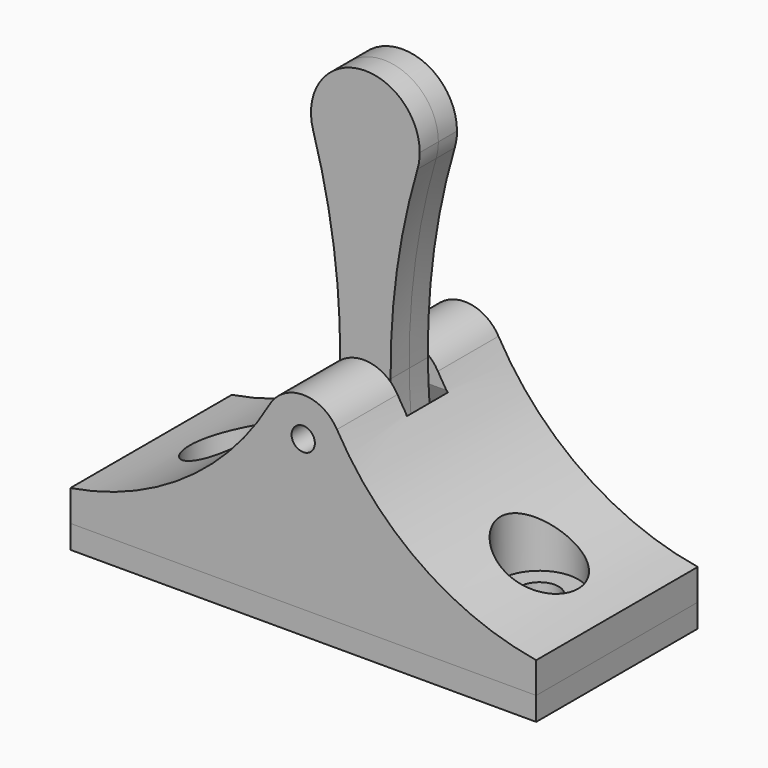
from build123d import *

# Parameters (mm, degrees)
F0_R          = 1.5
F1_DEPTH      = 3
F1_DEPTH_BACK = 3
F2_DEPTH      = 13
F2_DEPTH_BACK = 13
F3_W          = 11
F3_H          = 6.5
F4_DEPTH      = 25
F4_TAPER      = -22
F4_DEPTH_BACK = 25
F5_START      = -20
F3_W_2        = 60
F3_H_2        = 26
F3_R          = 5
F3_W_3        = 19
F3_H_3        = 13.5
F3_R_2        = 2.5
F5_DEPTH      = 3
F6_DEPTH      = 25
F7_DEPTH      = 17


# Not quite as in the source:
# - a feature names something its author has since deleted; it is built from what else it names


with BuildPart() as f1:
    # F0 (on Front) → F1 (new body, two sides)
    with BuildSketch(Plane.XZ) as f1_sk:
        with BuildLine():
            ThreePointArc((3.0397368307, -16), (4.3012352845, -14.3654093944), (4.75, -12.35))
            ThreePointArc((4.75, -12.35), (4.7300948444, -11.9156006874), (4.6705462051, -11.4848421267))
            ThreePointArc((4.6705462051, -11.4848421267), (0, -7.6), (-4.6705462051, -11.4848421267))
            ThreePointArc((-4.6705462051, -11.4848421267), (-4.4675249052, -13.9636050389), (-3.0397368307, -16))
            Line((-3.0397368307, -16), (3.0397368307, -16))
        make_face()
        with BuildLine():
            ThreePointArc((-4.6705462051, -11.4848421267), (0, -7.6), (4.6705462051, -11.4848421267))
            ThreePointArc((4.6705462051, -11.4848421267), (4.0724799807, -7.8080264222), (3.6360864347, -4.1085375916))
            ThreePointArc((3.6360864347, -4.1085375916), (0, -5.6765009603), (-3.6360864347, -4.1085375916))
            ThreePointArc((-3.6360864347, -4.1085375916), (-4.0724799807, -7.8080264222), (-4.6705462051, -11.4848421267))
        make_face()
        with BuildLine():
            ThreePointArc((-3.0397368307, -16), (0, -17.1), (3.0397368307, -16))
            Line((3.0397368307, -16), (-3.0397368307, -16))
        make_face()
        with BuildLine():
            ThreePointArc((-3.6360864347, -4.1085375916), (0, -5.6765009603), (3.6360864347, -4.1085375916))
            ThreePointArc((3.6360864347, -4.1085375916), (3.3676823781, -0.498156975), (3.2532612438, 3.1203781897))
            ThreePointArc((3.2532612438, 3.1203781897), (0, 4.3234990397), (-3.2532612438, 3.1203781897))
            ThreePointArc((-3.2532612438, 3.1203781897), (-3.3676823781, -0.498156975), (-3.6360864347, -4.1085375916))
        make_face()
        with Locations((0, -0.6765009603)):
            Circle(F0_R, mode=Mode.SUBTRACT)
        with BuildLine():
            ThreePointArc((-3.2532612438, 3.1203781897), (0, 4.3234990397), (3.2532612438, 3.1203781897))
            ThreePointArc((3.2532612438, 3.1203781897), (4.0582011416, 15.6996189973), (6.7145781542, 28.0215055695))
            ThreePointArc((6.7145781542, 28.0215055695), (0, 23), (-6.7145781542, 28.0215055695))
            ThreePointArc((-6.7145781542, 28.0215055695), (-4.0582011416, 15.6996189973), (-3.2532612438, 3.1203781897))
        make_face()
        with BuildLine():
            ThreePointArc((-6.7145781542, 28.0215055695), (0, 23), (6.7145781542, 28.0215055695))
            ThreePointArc((6.7145781542, 28.0215055695), (6.9282770975, 29.0005119008), (7, 30))
            ThreePointArc((7, 30), (-0.9994880992, 36.9282770975), (-6.7145781542, 28.0215055695))
        make_face()
    extrude(amount=F1_DEPTH)
    extrude(f1_sk.sketch, amount=-F1_DEPTH_BACK)


with BuildPart() as f2:
    # F0 (on Front) → F2 (new body, two sides)
    with BuildSketch(Plane.XZ) as f2_sk:
        with BuildLine():
            ThreePointArc((3.0397368307, -16), (4.3012352845, -14.3654093944), (4.75, -12.35))
            ThreePointArc((4.75, -12.35), (4.7300948444, -11.9156006874), (4.6705462051, -11.4848421267))
            ThreePointArc((4.6705462051, -11.4848421267), (0, -7.6), (-4.6705462051, -11.4848421267))
            ThreePointArc((-4.6705462051, -11.4848421267), (-4.4675249052, -13.9636050389), (-3.0397368307, -16))
            Line((-3.0397368307, -16), (3.0397368307, -16))
        make_face()
        with BuildLine():
            ThreePointArc((4.6705462051, -11.4848421267), (4.7300948444, -11.9156006874), (4.75, -12.35))
            ThreePointArc((4.75, -12.35), (4.3012352845, -14.3654093944), (3.0397368307, -16))
            Line((3.0397368307, -16), (30, -16))
            ThreePointArc((30, -16), (15.1577815574, -9.9967996829), (4.3401298873, 1.8060929577))
            ThreePointArc((4.3401298873, 1.8060929577), (4.8322173708, 0.607895895), (5, -0.6765009603))
            ThreePointArc((5, -0.6765009603), (4.6465273148, -2.5230609818), (3.6360864347, -4.1085375916))
            ThreePointArc((3.6360864347, -4.1085375916), (4.0724799807, -7.8080264222), (4.6705462051, -11.4848421267))
        make_face()
        with BuildLine():
            ThreePointArc((-4.6705462051, -11.4848421267), (0, -7.6), (4.6705462051, -11.4848421267))
            ThreePointArc((4.6705462051, -11.4848421267), (4.0724799807, -7.8080264222), (3.6360864347, -4.1085375916))
            ThreePointArc((3.6360864347, -4.1085375916), (0, -5.6765009603), (-3.6360864347, -4.1085375916))
            ThreePointArc((-3.6360864347, -4.1085375916), (-4.0724799807, -7.8080264222), (-4.6705462051, -11.4848421267))
        make_face()
        with BuildLine():
            Line((30, -16), (3.0397368307, -16))
            ThreePointArc((3.0397368307, -16), (0, -17.1), (-3.0397368307, -16))
            Line((-3.0397368307, -16), (-30, -16))
            Line((-30, -16), (-30, -20))
            Line((-30, -20), (30, -20))
            Line((30, -20), (30, -16))
        make_face()
        with BuildLine():
            ThreePointArc((-3.0397368307, -16), (0, -17.1), (3.0397368307, -16))
            Line((3.0397368307, -16), (-3.0397368307, -16))
        make_face()
        with BuildLine():
            ThreePointArc((-3.0397368307, -16), (-4.4675249052, -13.9636050389), (-4.6705462051, -11.4848421267))
            ThreePointArc((-4.6705462051, -11.4848421267), (-4.0724799807, -7.8080264222), (-3.6360864347, -4.1085375916))
            ThreePointArc((-3.6360864347, -4.1085375916), (-4.9649491778, -1.2674998285), (-4.3401298873, 1.8060929577))
            ThreePointArc((-4.3401298873, 1.8060929577), (-15.1577815574, -9.9967996829), (-30, -16))
            Line((-30, -16), (-3.0397368307, -16))
        make_face()
        with BuildLine():
            ThreePointArc((-3.6360864347, -4.1085375916), (0, -5.6765009603), (3.6360864347, -4.1085375916))
            ThreePointArc((3.6360864347, -4.1085375916), (3.3676823781, -0.498156975), (3.2532612438, 3.1203781897))
            ThreePointArc((3.2532612438, 3.1203781897), (0, 4.3234990397), (-3.2532612438, 3.1203781897))
            ThreePointArc((-3.2532612438, 3.1203781897), (-3.3676823781, -0.498156975), (-3.6360864347, -4.1085375916))
        make_face()
        with Locations((0, -0.6765009603)):
            Circle(F0_R, mode=Mode.SUBTRACT)
        with BuildLine():
            ThreePointArc((3.2532612438, 3.1203781897), (3.3676823781, -0.498156975), (3.6360864347, -4.1085375916))
            ThreePointArc((3.6360864347, -4.1085375916), (4.6465273148, -2.5230609818), (5, -0.6765009603))
            ThreePointArc((5, -0.6765009603), (4.8322173708, 0.607895895), (4.3401298873, 1.8060929577))
            ThreePointArc((4.3401298873, 1.8060929577), (3.85314594, 2.5099180902), (3.2532612438, 3.1203781897))
        make_face()
        with BuildLine():
            ThreePointArc((-4.3401298873, 1.8060929577), (-4.9649491778, -1.2674998285), (-3.6360864347, -4.1085375916))
            ThreePointArc((-3.6360864347, -4.1085375916), (-3.3676823781, -0.498156975), (-3.2532612438, 3.1203781897))
            ThreePointArc((-3.2532612438, 3.1203781897), (-3.85314594, 2.5099180902), (-4.3401298873, 1.8060929577))
        make_face()
    extrude(amount=F2_DEPTH)
    extrude(f2_sk.sketch, amount=-F2_DEPTH_BACK)

    # F3 (on Top) → F4 (cut, two sides)
    with BuildSketch(Plane.XY) as f4_sk:
        Rectangle(F3_W, F3_H)
    extrude(amount=-F4_DEPTH, taper=F4_TAPER, mode=Mode.SUBTRACT)
    extrude(f4_sk.sketch, amount=F4_DEPTH_BACK, mode=Mode.SUBTRACT)

    # F3 (on Top) → F6 (cut)
    with BuildSketch(Plane.XY):
        with Locations((-20, 0)):
            Circle(F3_R_2)
        with Locations((20, 0)):
            Circle(F3_R_2)
    extrude(amount=-F6_DEPTH, mode=Mode.SUBTRACT)

    # F3 (on Top) → F7 (cut)
    with BuildSketch(Plane.XY):
        with Locations((-20, 0)):
            Circle(F3_R)
        with Locations((-20, 0)):
            Circle(F3_R_2, mode=Mode.SUBTRACT)
        with Locations((20, 0)):
            Circle(F3_R)
        with Locations((20, 0)):
            Circle(F3_R_2, mode=Mode.SUBTRACT)
    extrude(amount=-F7_DEPTH, mode=Mode.SUBTRACT)


with BuildPart() as f5:
    # F3 (on Top) → F5 (new body)
    with BuildSketch(Plane.XY.offset(F5_START)):
        Rectangle(F3_W_2, F3_H_2)
        with Locations((-20, 0)):
            Circle(F3_R, mode=Mode.SUBTRACT)
        Rectangle(F3_W_3, F3_H_3, mode=Mode.SUBTRACT)
        with Locations((20, 0)):
            Circle(F3_R, mode=Mode.SUBTRACT)
        with Locations((20, 0)):
            Circle(F3_R)
        with Locations((20, 0)):
            Circle(F3_R_2, mode=Mode.SUBTRACT)
        with Locations((-20, 0)):
            Circle(F3_R)
        with Locations((-20, 0)):
            Circle(F3_R_2, mode=Mode.SUBTRACT)
    extrude(amount=-F5_DEPTH)


solid = Compound([f1.part, f2.part, f5.part])
